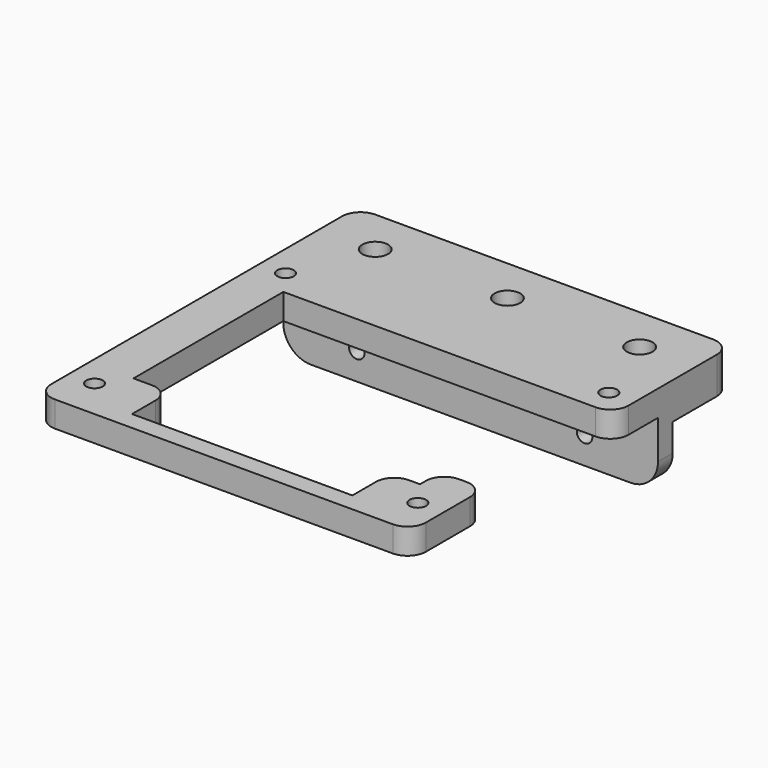
from build123d import *

# Parameters (mm, degrees)
F0_W      = 102
F0_H      = 84
F0_R      = 2.25
F0_W_2    = 78
F0_H_2    = 51
F1_DEPTH  = 15
F3_DEPTH  = 4
F4_W      = 12
F4_H      = 44
F4_W_2    = 60
F4_H_2    = 13
F5_DEPTH  = 15.001
F6_W      = 102
F6_H      = 84
F7_DEPTH  = 8
F8_W      = 102
F8_H      = 25
F8_R      = 2.125
F9_DEPTH  = 10
F10_R     = 3.5
F11_DEPTH = 5
F12_R     = 5
F13_W     = 102
F13_H     = 5
F14_DEPTH = 15
F15_R     = 2.125
F16_DEPTH = 25
F17_R     = 7.5


with BuildPart() as f1:
    # F0 (on Top) → F1 (new body)
    with BuildSketch(Plane.XY):
        with Locations((0, -1.5)):
            Rectangle(F0_W, F0_H)
        with Locations((-44, -32.5)):
            Circle(F0_R, mode=Mode.SUBTRACT)
        with Locations((44, -32.5)):
            Circle(F0_R, mode=Mode.SUBTRACT)
        with Locations((-44, 32.5)):
            Circle(F0_R, mode=Mode.SUBTRACT)
        Rectangle(F0_W_2, F0_H_2, mode=Mode.SUBTRACT)
        with Locations((44, 32.5)):
            Circle(F0_R, mode=Mode.SUBTRACT)
    extrude(amount=F1_DEPTH)

    # F2 (on face) → F3 (cut)
    with BuildSketch(Plane(origin=(0, 0, 0), x_dir=(1, 0, 0), z_dir=(0, 0, -1))):
        Polygon((-41.075, 30.8112504626), (-41.075, 34.1887495374), (-44, 35.8774990748), (-46.925, 34.1887495374), (-46.925, 30.8112504626), (-44, 29.1225009252), align=None)
        Polygon((41.075, 34.1887495374), (41.075, 30.8112504626), (44, 29.1225009252), (46.925, 30.8112504626), (46.925, 34.1887495374), (44, 35.8774990748), align=None)
        Polygon((41.075, -30.8112504626), (41.075, -34.1887495374), (44, -35.8774990748), (46.925, -34.1887495374), (46.925, -30.8112504626), (44, -29.1225009252), align=None)
        Polygon((-41.075, -34.1887495374), (-41.075, -30.8112504626), (-44, -29.1225009252), (-46.925, -30.8112504626), (-46.925, -34.1887495374), (-44, -35.8774990748), align=None)
    extrude(amount=-F3_DEPTH, mode=Mode.SUBTRACT)

    # F4 (on face) → F5 (cut, through all)
    with BuildSketch(Plane.XY.offset(15)):
        with Locations((45, 3.5)):
            Rectangle(F4_W, F4_H)
        with Locations((1, -32)):
            Rectangle(F4_W_2, F4_H_2)
    extrude(amount=-F5_DEPTH, mode=Mode.SUBTRACT)

    # F6 (on face) → F7 (cut)
    with BuildSketch(Plane.XY.offset(15)):
        with Locations((0, -1.5)):
            Rectangle(F6_W, F6_H)
    extrude(amount=-F7_DEPTH, mode=Mode.SUBTRACT)

    # F8 (on face) → F9 (join)
    with BuildSketch(Plane.XY.offset(7)):
        with Locations((0, 53)):
            Rectangle(F8_W, F8_H)
        with Locations((-36, 53)):
            Circle(F8_R, mode=Mode.SUBTRACT)
        with Locations((0, 53)):
            Circle(F8_R, mode=Mode.SUBTRACT)
        with Locations((36, 53)):
            Circle(F8_R, mode=Mode.SUBTRACT)
    extrude(amount=-F9_DEPTH)

    # F10 (on face) → F11 (cut)
    with BuildSketch(Plane.XY.offset(7)):
        with Locations((36, 53)):
            Circle(F10_R)
        with Locations((0, 53)):
            Circle(F10_R)
        with Locations((-36, 53)):
            Circle(F10_R)
    extrude(amount=-F11_DEPTH, mode=Mode.SUBTRACT)

    # F12
    f12_edges = [f1.edges().sort_by_distance(p)[0] for p in [
        (-51, -43.5, 3.5),
        (51, -43.5, 3.5),
        (51, 25.5, 3.5),
        (51, -18.5, 3.5),
        (39, -18.5, 3.5),
        (31, -25.5, 3.5),
        (-29, -25.5, 3.5),
        (-51, 65.5, 2),
        (51, 65.5, 2),
    ]]
    fillet(f12_edges, radius=F12_R)

    # F13 (on face) → F14 (join)
    with BuildSketch(Plane(origin=(0, 0, -3), x_dir=(1, 0, 0), z_dir=(0, 0, -1))):
        with Locations((0, -43)):
            Rectangle(F13_W, F13_H)
    extrude(amount=F14_DEPTH)

    # F15 (on face) → F16 (cut)
    with BuildSketch(Plane.XZ.offset(-40.5)):
        with Locations((-31, -10.5)):
            Circle(F15_R)
        with Locations((31, -10.5)):
            Circle(F15_R)
    extrude(amount=-F16_DEPTH, mode=Mode.SUBTRACT)

    # F17
    f17_edges = [f1.edges().sort_by_distance(p)[0] for p in [
        (-51, 43, -18),
        (51, 43, -18),
    ]]
    fillet(f17_edges, radius=F17_R)


solid = f1.part
